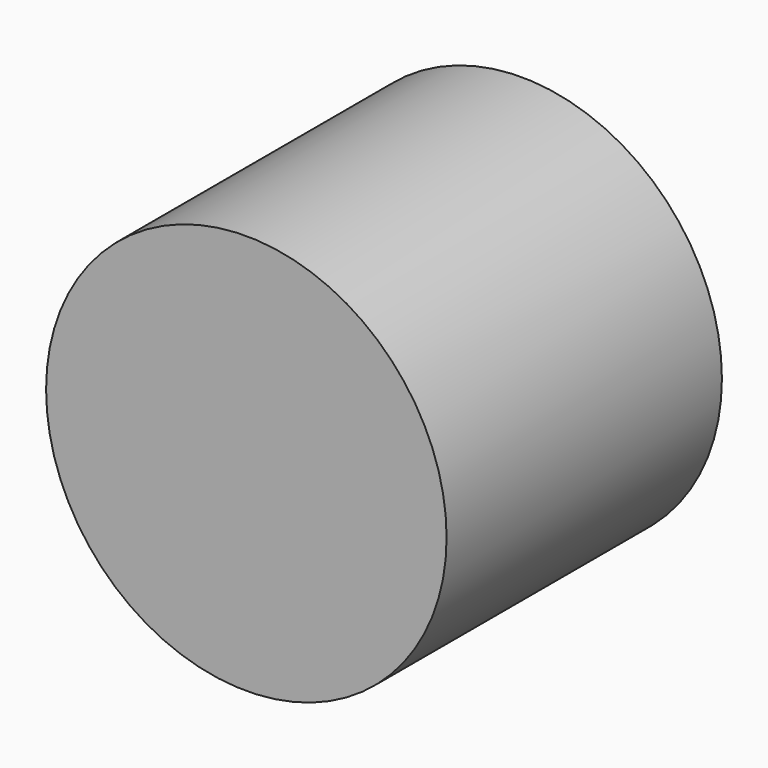
from build123d import *

# Parameters (mm, degrees)
F2_R     = 73.9013160002
F3_DEPTH = 127


# Not quite as in the source:
# - the program builds the solid bodies; features that only make, move or delete a surface that nothing else refers to are left out


with BuildPart() as f3:
    # F2 (on Front) → F3 (new body)
    with BuildSketch(Plane.XZ):
        Circle(F2_R)
    extrude(amount=F3_DEPTH)


solid = f3.part
